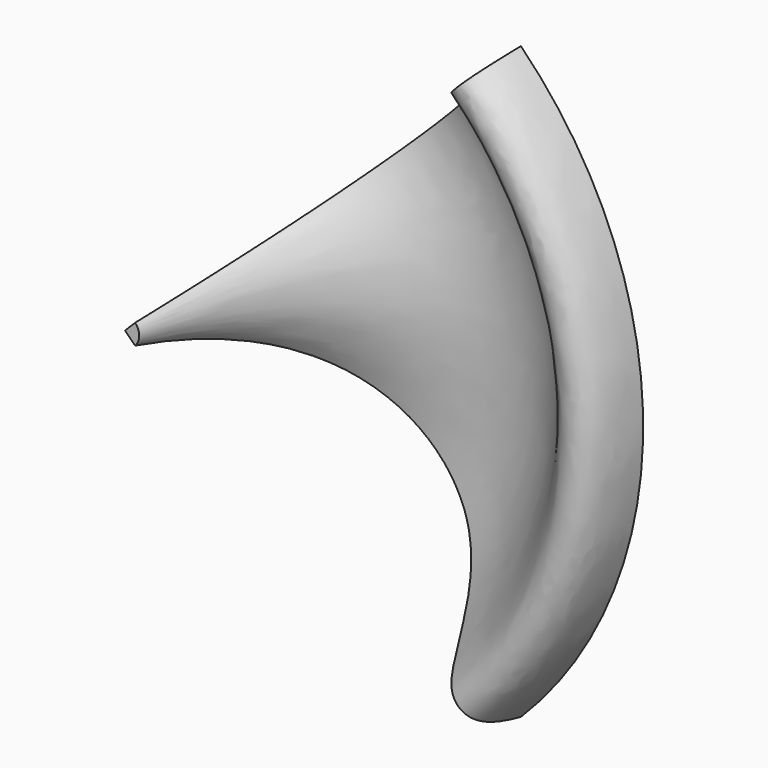
from build123d import *

# Parameters (mm, degrees)
F1_ANGLE_BACK = 45
F1_ANGLE      = 90


# Not quite as in the source:
# - ends of sketch curves that miss each other by under 0.0002 mm in the source are joined
# - the dataset's text gives a spline's control points without its knots; the knots are read off the source's solid


with BuildPart() as f1:
    # F0 (on Top) → F1 (revolve)
    with BuildSketch(Plane.XY, mode=Mode.PRIVATE) as f1_sk:
        with BuildLine():
            add(Edge.make_bspline(
                [(0, 0), (7.5545059517, 28.8444776088), (36.1764002964, 35.3689736788), (47.7648001273, 13.9484755375), (52.4236895144, 10.0726746023), (53.7804927516, 17.073170935)],
                knots=[0, 0, 0, 0, 0.4924352262, 0.8217214456, 1, 1, 1, 1], degree=3))
            Line((0, 0), (1.8908958035, 0))
            add(Edge.make_bspline(
                [(1.8908958035, 0), (2.8007279406, 3.3937484815), (4.9344372314, 9.5728823131), (8.7932893732, 16.7431514441), (13.1382071832, 21.9923778182), (17.6979466828, 25.4611056431), (22.2934713158, 27.4055123984), (26.0298084511, 27.9491983834), (28.8858165344, 27.8360778802), (30.938509042, 27.5000856383), (32.8801249341, 26.9356974704), (34.6787840721, 26.1692339077), (36.3384767665, 25.2167989691), (37.8828911261, 24.1011664468), (39.3213327108, 22.8492114001), (40.663818953, 21.4898167632), (41.9192385431, 20.0541620326), (43.0972916311, 18.5746913149), (44.2088154847, 17.0842928053), (45.2661848053, 15.6155781312), (46.1144882943, 14.435876141), (46.7820500831, 13.5337937602), (47.28106746, 12.8807669104), (47.7772682722, 12.25776991), (48.3026728516, 11.64367297), (48.8798577722, 11.0610104009), (49.4485707557, 10.6127430251), (50.0151397054, 10.3034854787), (50.5155894733, 10.1179935354), (51.0996941472, 10.0167453102), (51.7409141716, 10.0487923513), (52.3688822573, 10.2366777961), (52.9162234481, 10.5497937014), (53.3644644412, 10.9379948098), (53.8521276003, 11.5156479979), (54.319551773, 12.3276753891), (54.7820314633, 13.4942363777), (55.1950669257, 14.9223531848), (55.4506887983, 16.0844038811), (55.5749204327, 16.725383411)],
                knots=[0.0027062634, 0.0027062634, 0.0027062634, 0.0027062634, 0.0625, 0.125, 0.1875, 0.25, 0.3125, 0.375, 0.40625, 0.4375, 0.46875, 0.5, 0.53125, 0.5625, 0.59375, 0.625, 0.65625, 0.6875, 0.71875, 0.75, 0.78125, 0.796875, 0.8125, 0.828125, 0.84375, 0.859375, 0.875, 0.8828125, 0.890625, 0.8984375, 0.90625, 0.9140625, 0.921875, 0.9296875, 0.9375, 0.953125, 0.96875, 0.984375, 1, 1, 1, 1], degree=3))
            Line((55.5749204327, 16.725383411), (53.7804927516, 17.073170935))
        make_face()
    revolve(f1_sk.sketch.rotate(Axis((0, 20.3253012151, 0), (0, 1, 0)), -F1_ANGLE_BACK), axis=Axis((0, 20.3253012151, 0), (0, 1, 0)), revolution_arc=F1_ANGLE)


solid = f1.part
